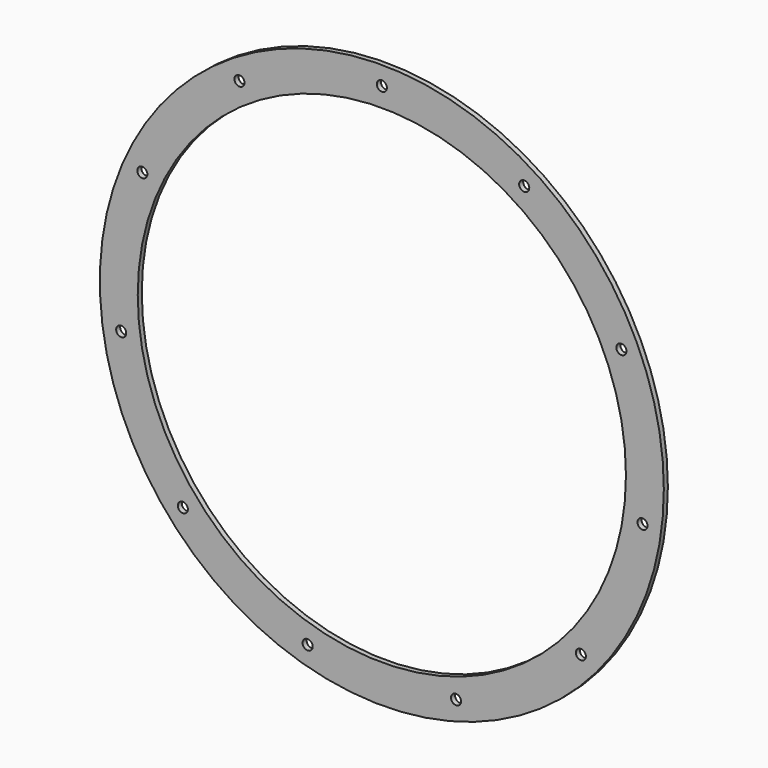
from build123d import *

# Parameters (mm, degrees)
F0_R            = 167.5
F0_R_2          = 145
F1_DEPTH        = 3
F2_R            = 3
F3_DEPTH        = 25
F3_COPIES_COUNT = 11


# Not quite as in the source:
# - a pattern or mirror of a feature is missing from the dataset's text; its kind, count and spacing are read off the source's solid


with BuildPart() as f1:
    # F0 (on Front) → F1 (new body)
    with BuildSketch(Plane.XZ):
        Circle(F0_R)
        Circle(F0_R_2, mode=Mode.SUBTRACT)
    extrude(amount=F1_DEPTH)

    # F2 (on face) → F3 (cut)
    with BuildSketch(Plane.XZ.offset(3)):
        with Locations((0, 156.4114242792)):
            Circle(F2_R)
    f3 = extrude(amount=-F3_DEPTH, mode=Mode.SUBTRACT)

    # F3_copies: F3 ×11 about axis
    f3_copies_axis = Axis((0, 0, 0), (0, 1, 0))
    for i in range(1, F3_COPIES_COUNT):
        add(f3.rotate(f3_copies_axis, i * 360 / F3_COPIES_COUNT), mode=Mode.SUBTRACT)


solid = f1.part
